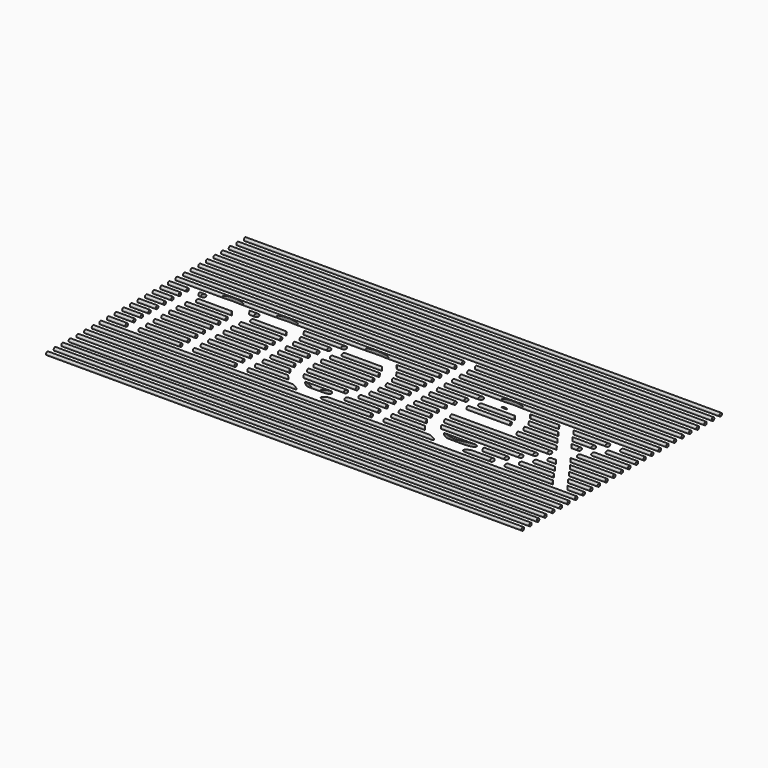
from build123d import *

# Parameters (mm, degrees)
F1_R         = 0.5
F3_TEXT_SIZE = 50.3937007874
F4_DEPTH     = 17.5


# Not quite as in the source:
# - Text() gives the source's letters only with a copy of the font that has no kerning and outlines rounded to 1/6400 em; it was checked with that copy


with BuildPart() as f2:
    # F2: sweep along a path in F0
    with BuildLine(Plane.XY) as f2_path:
        Line((-75, 69.1012981236), (75, 69.1012981236))
    # F1 (on Right) → F2 (sweep)
    with BuildSketch(Plane.YZ):
        with Locations((69.1012981236, 0)):
            Circle(F1_R)
        with Locations((66.1012981236, 0)):
            Circle(F1_R)
        with Locations((63.1012981236, 0)):
            Circle(F1_R)
        with Locations((60.1012981236, 0)):
            Circle(F1_R)
        with Locations((57.1012981236, 0)):
            Circle(F1_R)
        with Locations((54.1012981236, 0)):
            Circle(F1_R)
        with Locations((51.1012981236, 0)):
            Circle(F1_R)
        with Locations((48.1012981236, 0)):
            Circle(F1_R)
        with Locations((45.1012981236, 0)):
            Circle(F1_R)
        with Locations((42.1012981236, 0)):
            Circle(F1_R)
        with Locations((39.1012981236, 0)):
            Circle(F1_R)
        with Locations((36.1012981236, 0)):
            Circle(F1_R)
        with Locations((33.1012981236, 0)):
            Circle(F1_R)
        with Locations((30.1012981236, 0)):
            Circle(F1_R)
        with Locations((27.1012981236, 0)):
            Circle(F1_R)
        with Locations((24.1012981236, 0)):
            Circle(F1_R)
        with Locations((21.1012981236, 0)):
            Circle(F1_R)
        with Locations((18.1012981236, 0)):
            Circle(F1_R)
        with Locations((15.1012981236, 0)):
            Circle(F1_R)
        with Locations((12.1012981236, 0)):
            Circle(F1_R)
        with Locations((6.1012981236, 0)):
            Circle(F1_R)
        with Locations((3.1012981236, 0)):
            Circle(F1_R)
        with Locations((-8.8987018764, 0)):
            Circle(F1_R)
        with Locations((-5.8987018764, 0)):
            Circle(F1_R)
        with Locations((-2.8987018764, 0)):
            Circle(F1_R)
        Circle(F1_R)
        with Locations((9.1012981236, 0)):
            Circle(F1_R)
    sweep(path=f2_path.line)

    # F3 (on Top) → F4 (cut, symmetric)
    with BuildSketch(Plane.XY):
        with Locations((-73.5, 14.6012981236)):
            Text('molex', F3_TEXT_SIZE, font='Open Sans', text_align=(TextAlign.LEFT, TextAlign.BOTTOM))
    extrude(amount=F4_DEPTH, both=True, mode=Mode.SUBTRACT)


solid = f2.part
